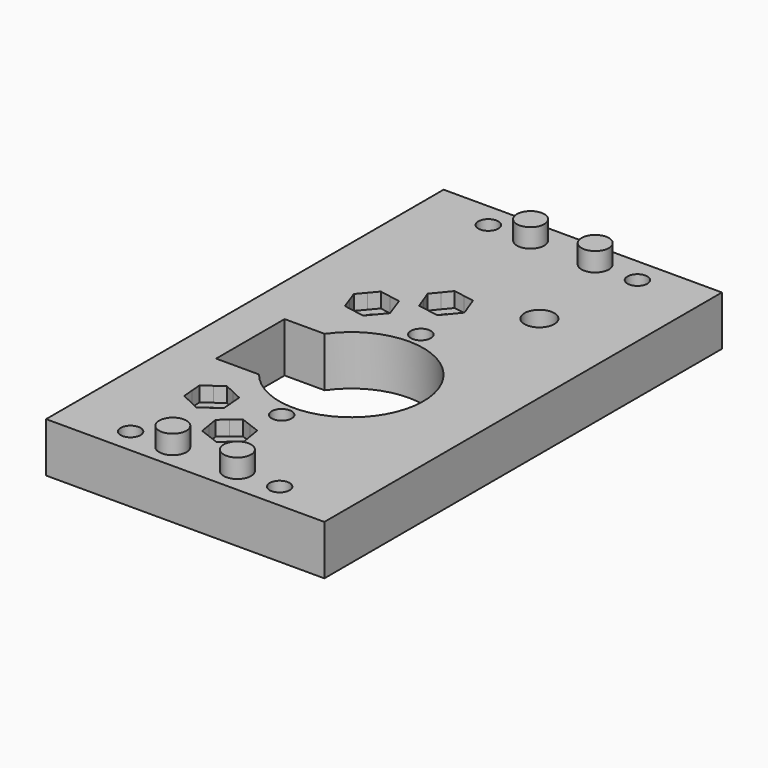
from build123d import *

# Parameters (mm, degrees)
F0_W      = 28
F0_H      = 50
F1_DEPTH  = 10
F3_DEPTH  = 10.001
F5_DEPTH  = 3.8
F6_R      = 4
F7_DEPTH  = 3
F10_R     = 2.05
F10_R_2   = 14.5
F11_DEPTH = 10.001
F12_R     = 2
F13_DEPTH = 10.001
F15_DEPTH = 10.001
F16_R     = 2
F16_R_2   = 2.9
F17_DEPTH = 25
F19_DEPTH = 3
F20_R     = 5.554436341
F21_DEPTH = 10
F22_R     = 3
F23_DEPTH = 25


with BuildPart() as f1:
    # F0 (on Top) → F1 (new body)
    with BuildSketch(Plane.XY):
        with Locations((-14, 25)):
            Rectangle(F0_W, F0_H)
    extrude(amount=F1_DEPTH)

    # F2 (on face) → F3 (cut, through all)
    with BuildSketch(Plane.XY.offset(10)):
        with BuildLine():
            ThreePointArc((-17, 45), (-15, 43), (-13, 45))
            Line((-13, 45), (-17, 45))
        make_face()
        with BuildLine():
            Line((-17, 45), (-13, 45))
            ThreePointArc((-13, 45), (-15, 47), (-17, 45))
        make_face()
    extrude(amount=-F3_DEPTH, mode=Mode.SUBTRACT)

    # F4 (on face) → F5 (join)
    with BuildSketch(Plane.XY.offset(10)):
        with BuildLine():
            ThreePointArc((-9.25, 45), (-6.5, 42.25), (-3.75, 45))
            ThreePointArc((-3.75, 45), (-6.5, 47.75), (-9.25, 45))
        make_face()
    extrude(amount=F5_DEPTH)

    # F6 (on face) → F7 (cut)
    with BuildSketch(Plane(origin=(0, 0, 0), x_dir=(1, 0, 0), z_dir=(0, 0, -1))):
        with Locations((-15, -45)):
            Circle(F6_R)
    extrude(amount=-F7_DEPTH, mode=Mode.SUBTRACT)

    # F8: F1 across plane


with BuildPart() as f1_1:
    add(f1.part)
    add(f1.part.mirror(Plane.XZ))

    # F9: F1 across plane


with BuildPart() as f1_2:
    add(f1_1.part)
    add(f1_1.part.mirror(Plane.YZ))

    # F10 (on face) → F11 (cut, through all)
    with BuildSketch(Plane.XY.offset(10)):
        with Locations((-12.4303577468, -27.8085004538)):
            Circle(F10_R)
        with Locations((-3.0035621021, -35.0598804653)):
            Circle(F10_R)
        with Locations((0, -8.2297706977)):
            Circle(F10_R_2)
    extrude(amount=-F11_DEPTH, mode=Mode.SUBTRACT)

    # F12 (on face) → F13 (cut, through all)
    with BuildSketch(Plane.XY.offset(10)):
        with Locations((0, -25.7297706977)):
            Circle(F12_R)
        with Locations((0, 9.2702293023)):
            Circle(F12_R)
    extrude(amount=-F13_DEPTH, mode=Mode.SUBTRACT)

    # F14 (on face) → F15 (cut, through all)
    with BuildSketch(Plane.XY.offset(10)):
        with BuildLine():
            Line((-20, -17.2297706977), (-11.3688170009, -17.2297706977))
            ThreePointArc((-11.3688170009, -17.2297706977), (-14.4920886836, -8.7086919702), (-11.938210681, 0))
            Line((-11.938210681, 0), (-20, 0))
            Line((-20, 0), (-20, -17.2297706977))
        make_face()
    extrude(amount=-F15_DEPTH, mode=Mode.SUBTRACT)

    # F16 (on face) → F17 (cut)
    with BuildSketch(Plane.XY.offset(10)):
        with Locations((-12.577921219, 12.6898593464)):
            Circle(F16_R)
        with Locations((-3.5732606182, 20.0715383219)):
            Circle(F16_R)
        with Locations((-11.7482841015, 30.8276228607)):
            Circle(F16_R_2)
    extrude(amount=-F17_DEPTH, mode=Mode.SUBTRACT)

    # F18 (on face) → F19 (cut)
    with BuildSketch(Plane.XY.offset(10)):
        with BuildLine():
            ThreePointArc((-10.2940314446, -30.890481948), (-9.1081804763, -29.5479366221), (-8.6803577468, -27.8085004538))
            ThreePointArc((-8.6803577468, -27.8085004538), (-8.683549751, -27.6538077178), (-8.6931203295, -27.499378331))
            ThreePointArc((-8.6931203295, -27.499378331), (-9.348376277, -25.6721741164), (-10.8294466879, -24.4173968309))
            ThreePointArc((-10.8294466879, -24.4173968309), (-12.7394799346, -24.0712630419), (-14.5666841389, -24.726519022))
            ThreePointArc((-14.5666841389, -24.726519022), (-15.8214613903, -26.2075894384), (-16.1675951564, -28.1176226698))
            ThreePointArc((-16.1675951564, -28.1176226698), (-15.51233919, -29.9448268296), (-14.0312688057, -31.1996040768))
            ThreePointArc((-14.0312688057, -31.1996040768), (-12.1212356135, -31.5457378703), (-10.2940314446, -30.890481948))
        make_face()
        with BuildLine():
            ThreePointArc((-8.6931203295, -27.499378331), (-8.683549751, -27.6538077178), (-8.6803577468, -27.8085004538))
            ThreePointArc((-8.6803577468, -27.8085004538), (-9.1081804763, -29.5479366221), (-10.2940314446, -30.890481948))
            Line((-10.2940314446, -30.890481948), (-8.5146485687, -29.6570733177))
            Line((-8.5146485687, -29.6570733177), (-8.6931203295, -27.499378331))
        make_face()
        with BuildLine():
            ThreePointArc((-10.8294466879, -24.4173968309), (-9.348376277, -25.6721741164), (-8.6931203295, -27.499378331))
            Line((-8.6931203295, -27.499378331), (-8.8715920969, -25.3416832638))
            Line((-8.8715920969, -25.3416832638), (-10.8294466879, -24.4173968309))
        make_face()
        with BuildLine():
            Line((-12.0734142186, -32.1238905078), (-10.2940314446, -30.890481948))
            ThreePointArc((-10.2940314446, -30.890481948), (-12.1212356135, -31.5457378703), (-14.0312688057, -31.1996040768))
            Line((-14.0312688057, -31.1996040768), (-12.0734142186, -32.1238905078))
        make_face()
        with BuildLine():
            ThreePointArc((-14.5666841389, -24.726519022), (-12.7394799346, -24.0712630419), (-10.8294466879, -24.4173968309))
            Line((-10.8294466879, -24.4173968309), (-12.7873012749, -23.4931103999))
            Line((-12.7873012749, -23.4931103999), (-14.5666841389, -24.726519022))
        make_face()
        with BuildLine():
            Line((-15.9891233967, -30.2753176439), (-14.0312688057, -31.1996040768))
            ThreePointArc((-14.0312688057, -31.1996040768), (-15.51233919, -29.9448268296), (-16.1675951564, -28.1176226698))
            Line((-16.1675951564, -28.1176226698), (-15.9891233967, -30.2753176439))
        make_face()
        with BuildLine():
            ThreePointArc((-16.1675951564, -28.1176226698), (-15.8214613903, -26.2075894384), (-14.5666841389, -24.726519022))
            Line((-14.5666841389, -24.726519022), (-16.3460669248, -25.95992759))
            Line((-16.3460669248, -25.95992759), (-16.1675951564, -28.1176226698))
        make_face()
        with BuildLine():
            ThreePointArc((-0.6247549112, -37.9588072233), (0.3863513899, -36.6633100761), (0.7464378979, -35.0598804653))
            ThreePointArc((0.7464378979, -35.0598804653), (0.733903899, -34.7535344349), (0.6963856897, -34.4492362663))
            ThreePointArc((0.6963856897, -34.4492362663), (-0.1046354718, -32.6810731187), (-1.6824217444, -31.5503095292))
            ThreePointArc((-1.6824217444, -31.5503095292), (-3.6142063621, -31.3599326835), (-5.3823693594, -32.1609537617))
            ThreePointArc((-5.3823693594, -32.1609537617), (-6.5131330001, -33.7387400064), (-6.7035098714, -35.6705248009))
            ThreePointArc((-6.7035098714, -35.6705248009), (-5.9024888018, -37.4386877272), (-4.3247027942, -38.5694512755))
            ThreePointArc((-4.3247027942, -38.5694512755), (-2.3929180607, -38.7598282831), (-0.6247549112, -37.9588072233))
        make_face()
        with BuildLine():
            ThreePointArc((0.6963856897, -34.4492362663), (0.733903899, -34.7535344349), (0.7464378979, -35.0598804653))
            ThreePointArc((0.7464378979, -35.0598804653), (0.3863513899, -36.6633100761), (-0.6247549112, -37.9588072233))
            Line((-0.6247549112, -37.9588072233), (1.048941297, -36.5854020812))
            Line((1.048941297, -36.5854020812), (0.6963856897, -34.4492362663))
        make_face()
        with BuildLine():
            ThreePointArc((-1.6824217444, -31.5503095292), (-0.1046354718, -32.6810731187), (0.6963856897, -34.4492362663))
            Line((0.6963856897, -34.4492362663), (0.3438300708, -32.3130703807))
            Line((0.3438300708, -32.3130703807), (-1.6824217444, -31.5503095292))
        make_face()
        with BuildLine():
            Line((-2.298450876, -39.3322121657), (-0.6247549112, -37.9588072233))
            ThreePointArc((-0.6247549112, -37.9588072233), (-2.3929180607, -38.7598282831), (-4.3247027942, -38.5694512755))
            Line((-4.3247027942, -38.5694512755), (-2.298450876, -39.3322121657))
        make_face()
        with BuildLine():
            ThreePointArc((-5.3823693594, -32.1609537617), (-3.6142063621, -31.3599326835), (-1.6824217444, -31.5503095292))
            Line((-1.6824217444, -31.5503095292), (-3.7086733282, -30.7875487648))
            Line((-3.7086733282, -30.7875487648), (-5.3823693594, -32.1609537617))
        make_face()
        with BuildLine():
            Line((-6.350954275, -37.8066905498), (-4.3247027942, -38.5694512755))
            ThreePointArc((-4.3247027942, -38.5694512755), (-5.9024888018, -37.4386877272), (-6.7035098714, -35.6705248009))
            Line((-6.7035098714, -35.6705248009), (-6.350954275, -37.8066905498))
        make_face()
        with BuildLine():
            ThreePointArc((-6.7035098714, -35.6705248009), (-6.5131330001, -33.7387400064), (-5.3823693594, -32.1609537617))
            Line((-5.3823693594, -32.1609537617), (-7.0560655012, -33.5343588494))
            Line((-7.0560655012, -33.5343588494), (-6.7035098714, -35.6705248009))
        make_face()
        with BuildLine():
            ThreePointArc((-9.7119539354, 10.2714442602), (-9.0558566744, 11.4023962039), (-8.827921219, 12.6898593464))
            ThreePointArc((-8.827921219, 12.6898593464), (-8.8839922837, 13.3359158612), (-9.0505286965, 13.9626523351))
            ThreePointArc((-9.0505286965, 13.9626523351), (-10.1595061384, 15.5558266347), (-11.9164959132, 16.3810673553))
            ThreePointArc((-11.9164959132, 16.3810673553), (-13.8507141383, 16.2172518939), (-15.4438885169, 15.1082744157))
            ThreePointArc((-15.4438885169, 15.1082744157), (-16.269129236, 13.3512846071), (-16.1053137706, 11.4170664382))
            ThreePointArc((-16.1053137706, 11.4170664382), (-14.9963363324, 9.8238920856), (-13.2393465249, 8.9986513375))
            ThreePointArc((-13.2393465249, 8.9986513375), (-11.3051283101, 9.1624667951), (-9.7119539354, 10.2714442602))
        make_face()
        with BuildLine():
            ThreePointArc((-9.0505286965, 13.9626523351), (-8.8839922837, 13.3359158612), (-8.827921219, 12.6898593464))
            ThreePointArc((-8.827921219, 12.6898593464), (-9.0558566744, 11.4023962039), (-9.7119539354, 10.2714442602))
            Line((-9.7119539354, 10.2714442602), (-8.3156813312, 11.9261112606))
            Line((-8.3156813312, 11.9261112606), (-9.0505286965, 13.9626523351))
        make_face()
        with BuildLine():
            ThreePointArc((-11.9164959132, 16.3810673553), (-10.1595061384, 15.5558266347), (-9.0505286965, 13.9626523351))
            Line((-9.0505286965, 13.9626523351), (-9.7853760307, 15.9991933234))
            Line((-9.7853760307, 15.9991933234), (-11.9164959132, 16.3810673553))
        make_face()
        with BuildLine():
            Line((-11.1082265195, 8.6167772836), (-9.7119539354, 10.2714442602))
            ThreePointArc((-9.7119539354, 10.2714442602), (-11.3051283101, 9.1624667951), (-13.2393465249, 8.9986513375))
            Line((-13.2393465249, 8.9986513375), (-11.1082265195, 8.6167772836))
        make_face()
        with BuildLine():
            ThreePointArc((-15.4438885169, 15.1082744157), (-13.8507141383, 16.2172518939), (-11.9164959132, 16.3810673553))
            Line((-11.9164959132, 16.3810673553), (-14.0476159186, 16.7629414092))
            Line((-14.0476159186, 16.7629414092), (-15.4438885169, 15.1082744157))
        make_face()
        with BuildLine():
            Line((-15.3704664073, 9.3805253694), (-13.2393465249, 8.9986513375))
            ThreePointArc((-13.2393465249, 8.9986513375), (-14.9963363324, 9.8238920856), (-16.1053137706, 11.4170664382))
            Line((-16.1053137706, 11.4170664382), (-15.3704664073, 9.3805253694))
        make_face()
        with BuildLine():
            ThreePointArc((-16.1053137706, 11.4170664382), (-16.269129236, 13.3512846071), (-15.4438885169, 15.1082744157))
            Line((-15.4438885169, 15.1082744157), (-16.8401611069, 13.4536074322))
            Line((-16.8401611069, 13.4536074322), (-16.1053137706, 11.4170664382))
        make_face()
        with BuildLine():
            ThreePointArc((-0.6773508715, 17.6890592058), (-0.0432350127, 18.8060663843), (0.1767393818, 20.0715383219))
            ThreePointArc((0.1767393818, 20.0715383219), (0.1165671942, 20.7406203163), (-0.0620183329, 21.3882302427))
            ThreePointArc((-0.0620183329, 21.3882302427), (-1.1907815138, 22.9674480783), (-2.957928008, 23.7707092802))
            ThreePointArc((-2.957928008, 23.7707092802), (-4.8899524085, 23.5827806561), (-6.4691703134, 22.4540175007))
            ThreePointArc((-6.4691703134, 22.4540175007), (-7.2724315792, 20.6868709158), (-7.084502922, 18.7548464508))
            ThreePointArc((-7.084502922, 18.7548464508), (-5.955739677, 17.1756285281), (-4.1885930596, 16.3723673355))
            ThreePointArc((-4.1885930596, 16.3723673355), (-2.2565687098, 16.560296032), (-0.6773508715, 17.6890592058))
        make_face()
        with BuildLine():
            ThreePointArc((-0.0620183329, 21.3882302427), (0.1165671942, 20.7406203163), (0.1767393818, 20.0715383219))
            ThreePointArc((0.1767393818, 20.0715383219), (-0.0432350127, 18.8060663843), (-0.6773508715, 17.6890592058))
            Line((-0.6773508715, 17.6890592058), (0.6981740932, 19.3610135117))
            Line((0.6981740932, 19.3610135117), (-0.0620183329, 21.3882302427))
        make_face()
        with BuildLine():
            ThreePointArc((-2.957928008, 23.7707092802), (-1.1907815138, 22.9674480783), (-0.0620183329, 21.3882302427))
            Line((-0.0620183329, 21.3882302427), (-0.8222107268, 23.4154468875))
            Line((-0.8222107268, 23.4154468875), (-2.957928008, 23.7707092802))
        make_face()
        with BuildLine():
            Line((-2.0528757981, 16.0171049461), (-0.6773508715, 17.6890592058))
            ThreePointArc((-0.6773508715, 17.6890592058), (-2.2565687098, 16.560296032), (-4.1885930596, 16.3723673355))
            Line((-4.1885930596, 16.3723673355), (-2.0528757981, 16.0171049461))
        make_face()
        with BuildLine():
            ThreePointArc((-6.4691703134, 22.4540175007), (-4.8899524085, 23.5827806561), (-2.957928008, 23.7707092802))
            Line((-2.957928008, 23.7707092802), (-5.0936454382, 24.1259716978))
            Line((-5.0936454382, 24.1259716978), (-6.4691703134, 22.4540175007))
        make_face()
        with BuildLine():
            Line((-6.3243105096, 16.7276297563), (-4.1885930596, 16.3723673355))
            ThreePointArc((-4.1885930596, 16.3723673355), (-5.955739677, 17.1756285281), (-7.084502922, 18.7548464508))
            Line((-7.084502922, 18.7548464508), (-6.3243105096, 16.7276297563))
        make_face()
        with BuildLine():
            ThreePointArc((-7.084502922, 18.7548464508), (-7.2724315792, 20.6868709158), (-6.4691703134, 22.4540175007))
            Line((-6.4691703134, 22.4540175007), (-7.8446953296, 20.7820631322))
            Line((-7.8446953296, 20.7820631322), (-7.084502922, 18.7548464508))
        make_face()
    extrude(amount=-F19_DEPTH, mode=Mode.SUBTRACT)

    # F20 (on face) → F21 (join)
    with BuildSketch(Plane.XY.offset(10)):
        with Locations((-11.7482841015, 30.8276228607)):
            Circle(F20_R)
    extrude(amount=-F21_DEPTH)

    # F22 (on face) → F23 (cut)
    with BuildSketch(Plane.XY.offset(10)):
        with Locations((11.1674116924, 25.1295231283)):
            Circle(F22_R)
    extrude(amount=-F23_DEPTH, mode=Mode.SUBTRACT)


solid = f1_2.part
